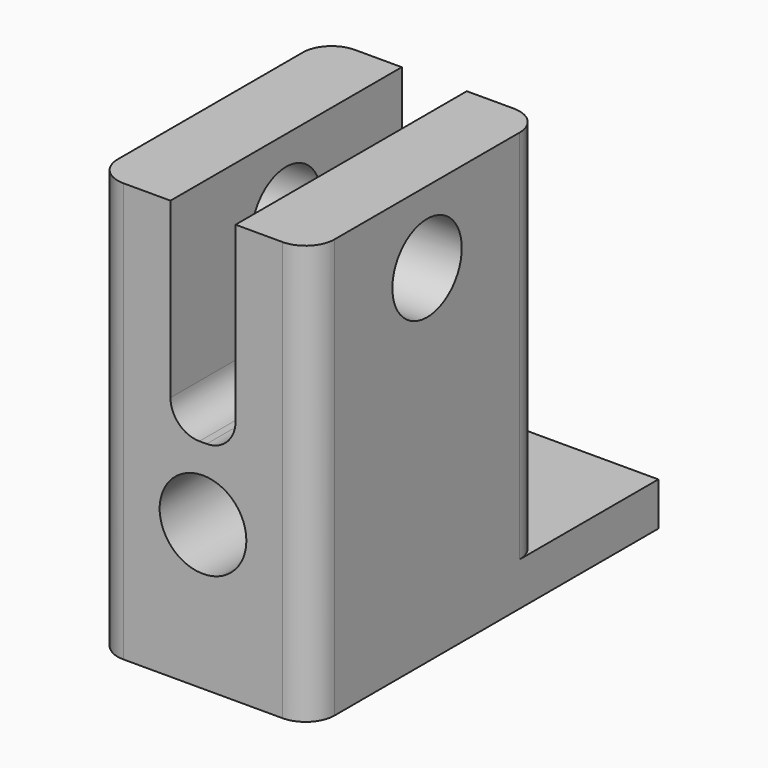
from build123d import *

# Parameters (mm, degrees)
F0_W          = 15
F0_H          = 20
F1_DEPTH      = 26
F2_R          = 3
F3_DEPTH      = 10.001
F3_DEPTH_BACK = 10.001
F4_R          = 3
F5_DEPTH      = 7.501
F5_DEPTH_BACK = 7.501
F6_W          = 4.5
F6_H          = 14
F7_DEPTH      = 10.001
F7_DEPTH_BACK = 10.001
F8_W          = 15
F8_H          = 30
F9_DEPTH      = 3
F10_R         = 2


# Not quite as in the source:
# - two fillets or chamfers of one size are made in one step
# - a feature names something its author has since deleted; it is built from what else it names


with BuildPart() as f1:
    # F0 (on Top) → F1 (new body)
    with BuildSketch(Plane.XY):
        Rectangle(F0_W, F0_H)
    extrude(amount=F1_DEPTH)

    # F2 (on Front) → F3 (cut, two sides)
    with BuildSketch(Plane.XZ) as f3_sk:
        with Locations((0, 7)):
            Circle(F2_R)
    extrude(amount=-F3_DEPTH, mode=Mode.SUBTRACT)
    extrude(f3_sk.sketch, amount=F3_DEPTH_BACK, mode=Mode.SUBTRACT)

    # F4 (on Right) → F5 (cut, two sides)
    with BuildSketch(Plane.YZ) as f5_sk:
        with Locations((0, 21)):
            Circle(F4_R)
    extrude(amount=-F5_DEPTH, mode=Mode.SUBTRACT)
    extrude(f5_sk.sketch, amount=F5_DEPTH_BACK, mode=Mode.SUBTRACT)

    # F6 (on Front) → F7 (cut, two sides)
    with BuildSketch(Plane.XZ) as f7_sk:
        with Locations((0, 19)):
            Rectangle(F6_W, F6_H)
    extrude(amount=-F7_DEPTH, mode=Mode.SUBTRACT)
    extrude(f7_sk.sketch, amount=F7_DEPTH_BACK, mode=Mode.SUBTRACT)

    # F8 (on face) → F9 (join)
    with BuildSketch(Plane(origin=(0, 0, 0), x_dir=(1, 0, 0), z_dir=(0, 0, -1))):
        with Locations((0, -5)):
            Rectangle(F8_W, F8_H)
    extrude(amount=F9_DEPTH)

    # F10
    f10_edges = [f1.edges().sort_by_distance(p)[0] for p in [
        (7.5, -10, 11.5),
        (-7.5, -10, 11.5),
        (-7.5, 10, 13),
        (7.5, 10, 13),
        (2.25, 0, 12),
        (-2.25, 0, 12),
    ]]
    fillet(f10_edges, radius=F10_R)


solid = f1.part
